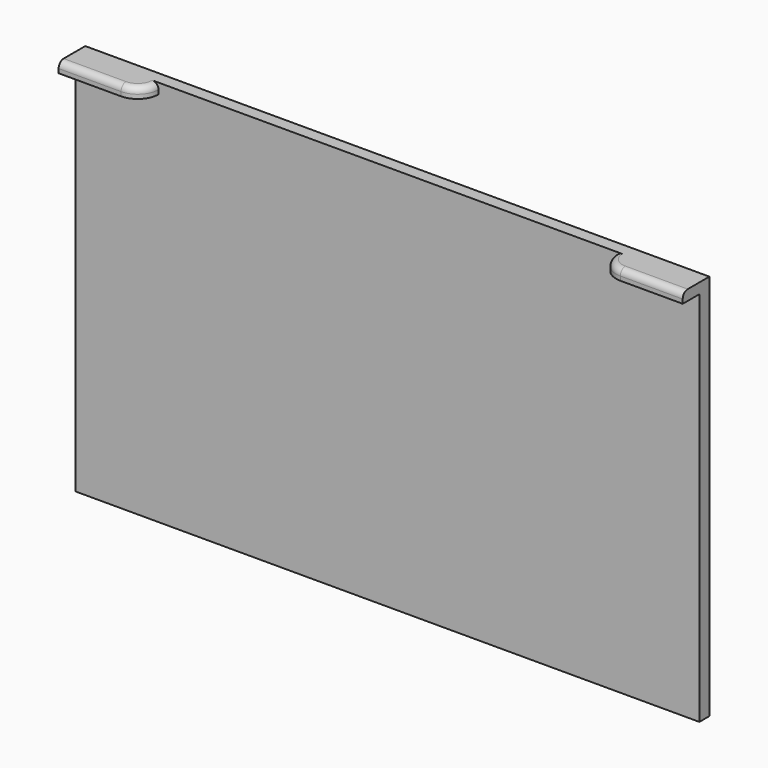
from build123d import *

# Parameters (mm, degrees)
F0_W     = 150
F0_H     = 93
F1_DEPTH = 3
F2_W     = 20
F2_H     = 2.5
F3_DEPTH = 5
F4_R     = 4.99999
F5_R     = 1.5


# Not quite as in the source:
# - a fillet or chamfer is up to 0.001 mm smaller than in the source, because OpenCascade refuses the exact size


with BuildPart() as f1:
    # F0 (on Front) → F1 (new body)
    with BuildSketch(Plane.XZ):
        with Locations((75, 46.5)):
            Rectangle(F0_W, F0_H)
    extrude(amount=F1_DEPTH)

    # F2 (on face) → F3 (join)
    with BuildSketch(Plane.XZ.offset(3)):
        with Locations((10, 91.75)):
            Rectangle(F2_W, F2_H)
        with Locations((140, 91.75)):
            Rectangle(F2_W, F2_H)
    extrude(amount=F3_DEPTH)

    # F4 (radius 5 in the source; OpenCascade refuses exactly that, so slightly less here)
    f4_edges = [f1.edges().sort_by_distance(p)[0] for p in [
        (20, -8, 91.75),
        (130, -8, 91.75),
    ]]
    fillet(f4_edges, radius=F4_R)

    # F5
    f5_edges = [f1.edges().sort_by_distance(p)[0] for p in [
        (7.500005, -8, 93),
        (142.499995, -8, 93),
    ]]
    fillet(f5_edges, radius=F5_R)


solid = f1.part
